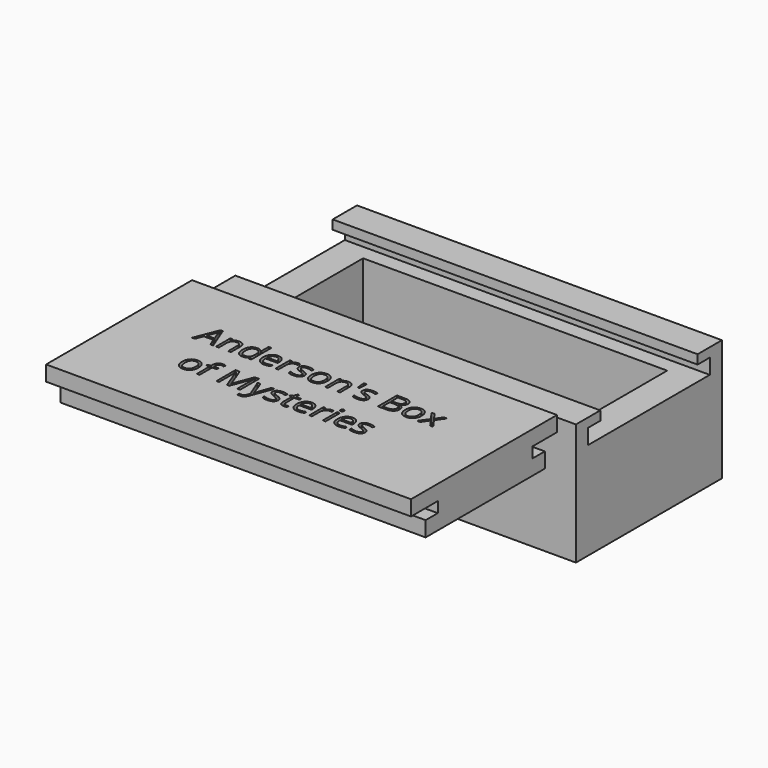
from build123d import *

# Parameters (mm, degrees)
F0_W         = 120
F0_H         = 60
F1_DEPTH     = 40
F2_W         = 100
F2_H         = 40
F3_DEPTH     = 30
F5_DEPTH     = 120
F7_DEPTH     = 120
F8_TEXT_SIZE = 10.9551523451
F9_DEPTH     = 3


# Not quite as in the source:
# - Text() gives the source's letters only with a copy of the font that has no kerning and outlines rounded to 1/6400 em; it was checked with that copy


with BuildPart() as f1:
    # F0 (on Top) → F1 (new body)
    with BuildSketch(Plane.XY):
        with Locations((60, 30)):
            Rectangle(F0_W, F0_H)
    extrude(amount=F1_DEPTH)

    # F2 (on face) → F3 (cut)
    with BuildSketch(Plane.XY.offset(40)):
        with Locations((60, 30)):
            Rectangle(F2_W, F2_H)
    extrude(amount=-F3_DEPTH, mode=Mode.SUBTRACT)

    # F4 (on face) → F5 (cut)
    with BuildSketch(Plane(origin=(0, 0, 0), x_dir=(0, -1, 0), z_dir=(-1, 0, 0))):
        Polygon((-50, 37), (-55, 37), (-55, 32), (-5, 32), (-5, 37), (-10, 37), (-10, 40), (-50, 40), align=None)
    extrude(amount=-F5_DEPTH, mode=Mode.SUBTRACT)


with BuildPart() as f7:
    # F6 (on Right) → F7 (new body)
    with BuildSketch(Plane.YZ):
        Polygon((-12.7981972694, 32.4089289606), (-12.7981972694, 37.4089289606), (-17.7981972694, 37.4089289606), (-17.7981972694, 40.9089289606), (-7.7981972694, 40.9089289606), (-7.7981972694, 45.9089289606), (-67.7981972694, 45.9089289606), (-67.7981972694, 40.9089289606), (-56.7981972694, 40.9089289606), (-56.7981972694, 37.4089289606), (-61.7981972694, 37.4089289606), (-61.7981972694, 32.4089289606), align=None)
    extrude(amount=F7_DEPTH)

    # F8 (on face) → F9 (cut)
    with BuildSketch(Plane.XY.offset(45.9089289606)):
        with Locations((20, -32.7981972694)):
            Text("Anderson's Box", F8_TEXT_SIZE, font='Open Sans', text_align=(TextAlign.LEFT, TextAlign.BOTTOM))
        with Locations((25.6932557343, -47.6972044588)):
            Text('of Mysteries', F8_TEXT_SIZE, font='Open Sans', text_align=(TextAlign.LEFT, TextAlign.BOTTOM))
    extrude(amount=-F9_DEPTH, mode=Mode.SUBTRACT)


solid = Compound([f1.part, f7.part])
